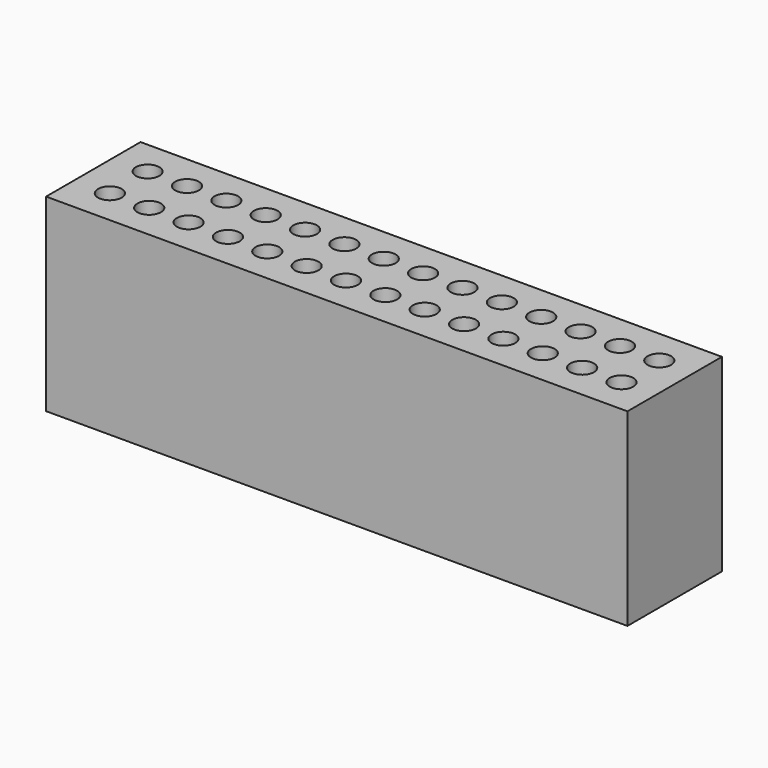
from build123d import *

# Parameters (mm, degrees)
F0_W     = 123.0850573922
F0_H     = 25
F0_R     = 2.5
F1_DEPTH = 40
F2_DEPTH = 40
F3_DEPTH = 5
F4_R     = 2.5


# Not quite as in the source:
# - a feature names something its author has since deleted; it is built from what else it names


with BuildPart() as f1:
    # F0 (on Top) → F1 (new body)
    with BuildSketch(Plane.XY):
        with Locations((18.6507174147, 3.4210662183)):
            Rectangle(F0_W, F0_H)
        with Locations((-35.3918112814, -1.5789337817)):
            Circle(F0_R, mode=Mode.SUBTRACT)
        with Locations((-27.0588112814, -1.5789337817)):
            Circle(F0_R, mode=Mode.SUBTRACT)
        with Locations((-18.7258112814, -1.5789337817)):
            Circle(F0_R, mode=Mode.SUBTRACT)
        with Locations((-10.3928112814, -1.5789337817)):
            Circle(F0_R, mode=Mode.SUBTRACT)
        with Locations((-2.0598112814, -1.5789337817)):
            Circle(F0_R, mode=Mode.SUBTRACT)
        with Locations((6.2731887186, -1.5789337817)):
            Circle(F0_R, mode=Mode.SUBTRACT)
        with Locations((14.6061887186, -1.5789337817)):
            Circle(F0_R, mode=Mode.SUBTRACT)
        with Locations((22.9391887186, -1.5789337817)):
            Circle(F0_R, mode=Mode.SUBTRACT)
        with Locations((31.2721887186, -1.5789337817)):
            Circle(F0_R, mode=Mode.SUBTRACT)
        with Locations((39.6051887186, -1.5789337817)):
            Circle(F0_R, mode=Mode.SUBTRACT)
        with Locations((47.9381887186, -1.5789337817)):
            Circle(F0_R, mode=Mode.SUBTRACT)
        with Locations((56.2711887186, -1.5789337817)):
            Circle(F0_R, mode=Mode.SUBTRACT)
        with Locations((64.6041887186, -1.5789337817)):
            Circle(F0_R, mode=Mode.SUBTRACT)
        with Locations((72.9371887186, -1.5789337817)):
            Circle(F0_R, mode=Mode.SUBTRACT)
        with Locations((-35.3918112814, 8.4210662183)):
            Circle(F0_R, mode=Mode.SUBTRACT)
        with Locations((-27.0588112814, 8.4210662183)):
            Circle(F0_R, mode=Mode.SUBTRACT)
        with Locations((-18.7258112814, 8.4210662183)):
            Circle(F0_R, mode=Mode.SUBTRACT)
        with Locations((-10.3928112814, 8.4210662183)):
            Circle(F0_R, mode=Mode.SUBTRACT)
        with Locations((-2.0598112814, 8.4210662183)):
            Circle(F0_R, mode=Mode.SUBTRACT)
        with Locations((6.2731887186, 8.4210662183)):
            Circle(F0_R, mode=Mode.SUBTRACT)
        with Locations((14.6061887186, 8.4210662183)):
            Circle(F0_R, mode=Mode.SUBTRACT)
        with Locations((22.9391887186, 8.4210662183)):
            Circle(F0_R, mode=Mode.SUBTRACT)
        with Locations((31.2721887186, 8.4210662183)):
            Circle(F0_R, mode=Mode.SUBTRACT)
        with Locations((39.6051887186, 8.4210662183)):
            Circle(F0_R, mode=Mode.SUBTRACT)
        with Locations((47.9381887186, 8.4210662183)):
            Circle(F0_R, mode=Mode.SUBTRACT)
        with Locations((56.2711887186, 8.4210662183)):
            Circle(F0_R, mode=Mode.SUBTRACT)
        with Locations((64.6041887186, 8.4210662183)):
            Circle(F0_R, mode=Mode.SUBTRACT)
        with Locations((72.9371887186, 8.4210662183)):
            Circle(F0_R, mode=Mode.SUBTRACT)
        with Locations((-35.3918112814, 8.4210662183)):
            Circle(F0_R)
        with Locations((-27.0588112814, 8.4210662183)):
            Circle(F0_R)
        with Locations((-27.0588112814, -1.5789337817)):
            Circle(F0_R)
        with Locations((-35.3918112814, -1.5789337817)):
            Circle(F0_R)
    extrude(amount=-F1_DEPTH)

    # F0 (on Top) → F2 (cut)
    with BuildSketch(Plane.XY):
        with Locations((-35.3918112814, 8.4210662183)):
            Circle(F0_R)
        with Locations((-27.0588112814, 8.4210662183)):
            Circle(F0_R)
        with Locations((-18.7258112814, 8.4210662183)):
            Circle(F0_R)
        with Locations((-10.3928112814, 8.4210662183)):
            Circle(F0_R)
        with Locations((-2.0598112814, 8.4210662183)):
            Circle(F0_R)
        with Locations((6.2731887186, 8.4210662183)):
            Circle(F0_R)
        with Locations((14.6061887186, 8.4210662183)):
            Circle(F0_R)
        with Locations((22.9391887186, 8.4210662183)):
            Circle(F0_R)
        with Locations((31.2721887186, 8.4210662183)):
            Circle(F0_R)
        with Locations((39.6051887186, 8.4210662183)):
            Circle(F0_R)
        with Locations((47.9381887186, 8.4210662183)):
            Circle(F0_R)
        with Locations((56.2711887186, 8.4210662183)):
            Circle(F0_R)
        with Locations((64.6041887186, 8.4210662183)):
            Circle(F0_R)
        with Locations((72.9371887186, 8.4210662183)):
            Circle(F0_R)
    extrude(amount=-F2_DEPTH, mode=Mode.SUBTRACT)

    # F0 (on Top) → F3 (cut)
    with BuildSketch(Plane.XY):
        with Locations((-35.3918112814, -1.5789337817)):
            Circle(F0_R)
        with Locations((-27.0588112814, -1.5789337817)):
            Circle(F0_R)
    extrude(amount=-F3_DEPTH, mode=Mode.SUBTRACT)

    # F4
    f4_edges = [f1.edges().sort_by_distance(p)[0] for p in [
        (-37.891811, -1.578934, -5),
        (-29.558811, -1.578934, -5),
    ]]
    fillet(f4_edges, radius=F4_R)


solid = f1.part
